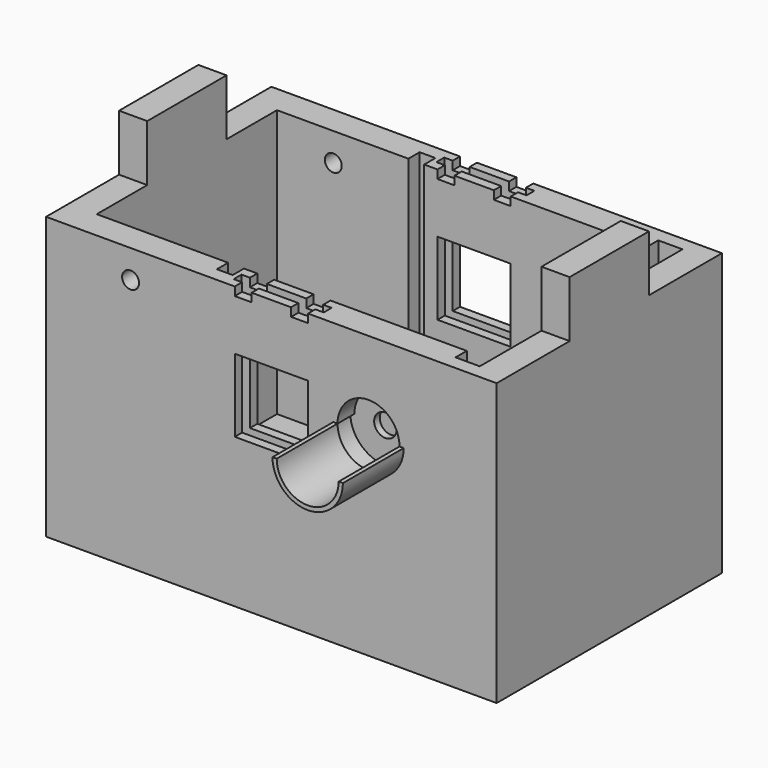
from build123d import *

# Parameters (mm, degrees)
F6_W      = 203.2
F6_H      = 127
F6_W_2    = 177.8
F6_H_2    = 101.6
F7_DEPTH  = 127
F8_DEPTH  = 6.35
F9_W      = 20.32
F9_H      = 4.445
F10_DEPTH = 63.5
F11_W     = 33.02
F11_H     = 33.02
F11_W_2   = 7.62
F11_H_2   = 3.81
F12_DEPTH = 127
F13_DEPTH = 12.7
F14_DEPTH = 9.525
F15_DEPTH = 34.29
F16_W     = 10.922
F16_H     = 6.35
F16_W_2   = 7.112
F17_DEPTH = 114.3
F18_W     = 12.7
F18_H     = 22.352
F19_DEPTH = 25.4
F20_R     = 3.81
F21_DEPTH = 127


# Not quite as in the source:
# - a variable given as a bare number and used for a length is read in inches; the dataset says mm whatever the document's units were


with BuildPart() as f7:
    # F6 (on Top) → F7 (new body)
    with BuildSketch(Plane.XY):
        with Locations((101.6, 63.5)):
            Rectangle(F6_W, F6_H)
        with Locations((101.6, 63.5)):
            Rectangle(F6_W_2, F6_H_2, mode=Mode.SUBTRACT)
    extrude(amount=F7_DEPTH)

    # F6 (on Top) → F8 (join)
    with BuildSketch(Plane.XY):
        with Locations((101.6, 63.5)):
            Rectangle(F6_W_2, F6_H_2)
    extrude(amount=F8_DEPTH)

    # F9 (on face) → F10 (cut)
    with BuildSketch(Plane.XY.offset(127)):
        with Locations((91.44, 6.35)):
            Rectangle(F9_W, F9_H)
        with Locations((111.76, 6.35)):
            Rectangle(F9_W, F9_H)
        with Locations((91.44, 120.65)):
            Rectangle(F9_W, F9_H)
        with Locations((111.76, 120.65)):
            Rectangle(F9_W, F9_H)
    extrude(amount=-F10_DEPTH, mode=Mode.SUBTRACT)

    # F11 (on face) → F12 (cut)
    with BuildSketch(Plane.XZ):
        with Locations((101.6, 83.82)):
            Rectangle(F11_W, F11_H)
        with Locations((88.9, 125.095)):
            Rectangle(F11_W_2, F11_H_2)
        with Locations((114.3, 125.095)):
            Rectangle(F11_W_2, F11_H_2)
    extrude(amount=-F12_DEPTH, mode=Mode.SUBTRACT)

    # F11 (on face) → F13 (cut)
    with BuildSketch(Plane.XZ):
        with BuildLine():
            Line((145.415, 87.63), (150.495, 87.63))
            ThreePointArc((150.495, 87.63), (145.415, 92.71), (140.335, 87.63))
            Line((140.335, 87.63), (145.415, 87.63))
        make_face()
        with BuildLine():
            ThreePointArc((140.335, 87.63), (145.415, 82.55), (150.495, 87.63))
            Line((150.495, 87.63), (145.415, 87.63))
            Line((145.415, 87.63), (140.335, 87.63))
        make_face()
    extrude(amount=-F13_DEPTH, mode=Mode.SUBTRACT)

    # F11 (on face) → F14 (cut)
    with BuildSketch(Plane.XZ):
        with BuildLine():
            Line((161.29, 87.63), (159.385, 87.63))
            ThreePointArc((159.385, 87.63), (145.415, 73.66), (131.445, 87.63))
            Line((131.445, 87.63), (129.54, 87.63))
            ThreePointArc((129.54, 87.63), (145.415, 71.755), (161.29, 87.63))
        make_face()
        with BuildLine():
            ThreePointArc((131.445, 87.63), (145.415, 73.66), (159.385, 87.63))
            Line((159.385, 87.63), (150.495, 87.63))
            ThreePointArc((150.495, 87.63), (145.415, 82.55), (140.335, 87.63))
            Line((140.335, 87.63), (131.445, 87.63))
        make_face()
        with BuildLine():
            Line((150.495, 87.63), (159.385, 87.63))
            ThreePointArc((159.385, 87.63), (145.415, 101.6), (131.445, 87.63))
            Line((131.445, 87.63), (140.335, 87.63))
            ThreePointArc((140.335, 87.63), (145.415, 92.71), (150.495, 87.63))
        make_face()
    extrude(amount=-F14_DEPTH, mode=Mode.SUBTRACT)

    # F16 (on face) → F17 (cut)
    with BuildSketch(Plane.XY.offset(127)):
        with Locations((185.039, 9.525)):
            Rectangle(F16_W, F16_H)
        with Locations((75.5226666667, 9.525)):
            Rectangle(F16_W_2, F16_H)
        with Locations((185.039, 117.475)):
            Rectangle(F16_W, F16_H)
        with Locations((75.5226666667, 117.475)):
            Rectangle(F16_W_2, F16_H)
    extrude(amount=-F17_DEPTH, mode=Mode.SUBTRACT)

    # F18 (on face) → F19 (join)
    with BuildSketch(Plane.XY.offset(127)):
        with Locations((6.35, 52.324)):
            Rectangle(F18_W, F18_H)
        with Locations((196.85, 52.324)):
            Rectangle(F18_W, F18_H)
        with Locations((196.85, 74.676)):
            Rectangle(F18_W, F18_H)
        with Locations((6.35, 74.676)):
            Rectangle(F18_W, F18_H)
    extrude(amount=F19_DEPTH)

    # F20 (on face) → F21 (cut)
    with BuildSketch(Plane.XZ):
        with Locations((38.1, 114.3)):
            Circle(F20_R)
    extrude(amount=-F21_DEPTH, mode=Mode.SUBTRACT)


with BuildPart() as f15:
    # F11 (on face) → F15 (new body)
    with BuildSketch(Plane.XZ):
        with BuildLine():
            Line((161.29, 87.63), (159.385, 87.63))
            ThreePointArc((159.385, 87.63), (145.415, 73.66), (131.445, 87.63))
            Line((131.445, 87.63), (129.54, 87.63))
            ThreePointArc((129.54, 87.63), (145.415, 71.755), (161.29, 87.63))
        make_face()
    extrude(amount=F15_DEPTH)


solid = Compound([f7.part, f15.part])
